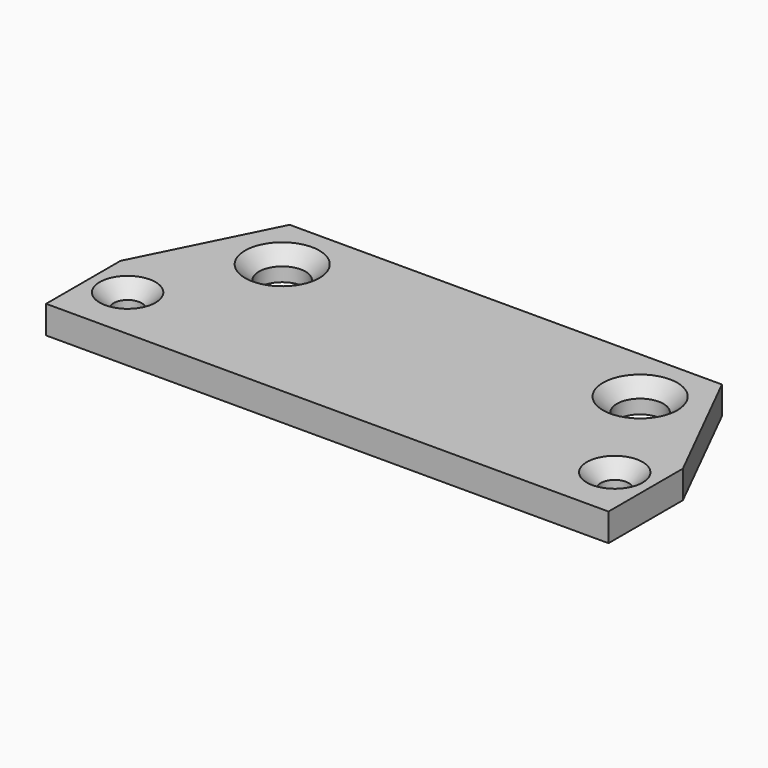
from build123d import *

# Parameters (mm, degrees)
F0_W     = 60.5
F0_H     = 10
F0_R     = 1.5
F0_R_2   = 2.5
F1_DEPTH = 3
F2_SIZE  = 1.5
F3_SIZE  = 1.5


# Not quite as in the source:
# - a feature names something its author has since deleted; it is built from what else it names


with BuildPart() as f1:
    # F0 (on Top) → F1 (new body)
    with BuildSketch(Plane.XY):
        with Locations((0, 54.5)):
            Rectangle(F0_W, F0_H)
        with Locations((-26.2, 55.4)):
            Circle(F0_R, mode=Mode.SUBTRACT)
        with Locations((26.2, 55.4)):
            Circle(F0_R, mode=Mode.SUBTRACT)
        Polygon((-23.25, 73.5), (-30.25, 59.5), (30.25, 59.5), (23.25, 73.5), align=None)
        with Locations((-19.25, 67.5)):
            Circle(F0_R_2, mode=Mode.SUBTRACT)
        with Locations((19.25, 67.5)):
            Circle(F0_R_2, mode=Mode.SUBTRACT)
    extrude(amount=F1_DEPTH)

    # F2
    f2_edges = [f1.edges().sort_by_distance(p)[0] for p in [
        (-27.7, 55.4, 3),
        (24.7, 55.4, 3),
    ]]
    chamfer(f2_edges, length=F2_SIZE)

    # F3
    f3_edges = [f1.edges().sort_by_distance(p)[0] for p in [
        (16.75, 67.5, 3),
        (-21.75, 67.5, 3),
    ]]
    chamfer(f3_edges, length=F3_SIZE)


solid = f1.part
